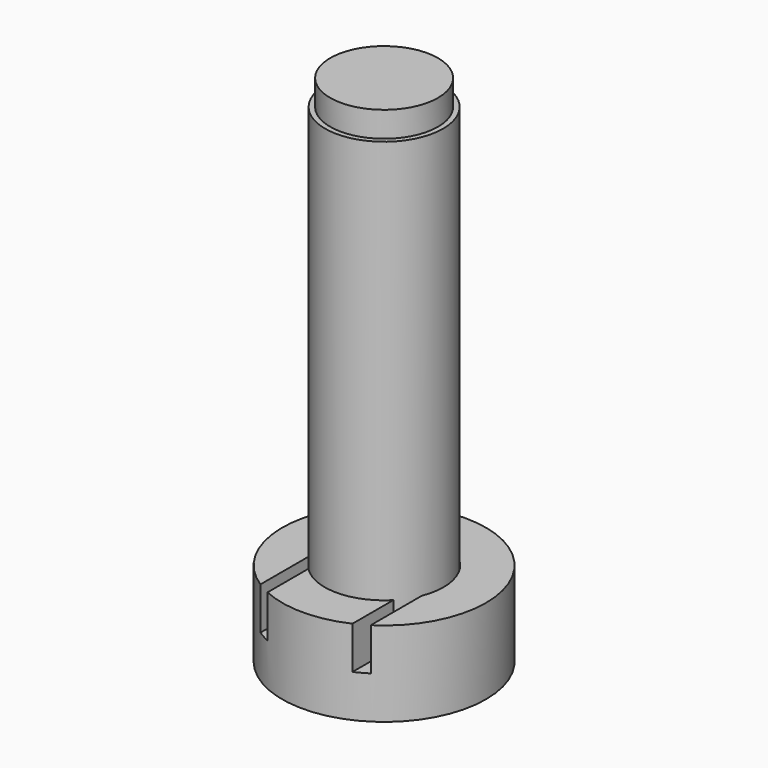
from build123d import *

# Parameters (mm, degrees)
F0_R      = 13.9
F0_R_2    = 8.7
F1_DEPTH  = 51.5
F2_R      = 12.7
F3_DEPTH  = 6
F4_R      = 10.3
F4_R_2    = 5.8
F5_DEPTH  = 2.05
F6_R      = 12.7
F7_DEPTH  = 6
F10_W     = 3
F10_H     = 25
F11_DEPTH = 10


with BuildPart() as f1:
    # F0 (on Top) → F1 (new body, symmetric)
    with BuildSketch(Plane.XY):
        Circle(F0_R)
        Circle(F0_R_2, mode=Mode.SUBTRACT)
    extrude(amount=F1_DEPTH, both=True)


with BuildPart() as f3:
    # F2 (on face) → F3 (new body)
    with BuildSketch(Plane.XY.offset(51.5)):
        Circle(F2_R)
    extrude(amount=F3_DEPTH)


with BuildPart() as f5:
    # F4 (on face) → F5 (new body)
    with BuildSketch(Plane(origin=(0, 0, -51.5), x_dir=(1, 0, 0), z_dir=(0, 0, -1))):
        Circle(F4_R)
        Circle(F4_R_2, mode=Mode.SUBTRACT)
    extrude(amount=F5_DEPTH)


with BuildPart() as f7:
    # F6 (on face) → F7 (new body)
    with BuildSketch(Plane(origin=(0, 0, -53.55), x_dir=(1, 0, 0), z_dir=(0, 0, -1))):
        Circle(F6_R)
    extrude(amount=F7_DEPTH)


with BuildPart() as f9:
    # F8 (on Front) → F9 (revolve)
    with BuildSketch(Plane.XZ):
        Polygon((5.7, -53.55), (5.7, -43.55), (0, -43.55), (0, -63.55), (24, -63.55), (24, -43.55), (14, -43.55), (14, -53.55), align=None)
    revolve(axis=Axis((0, 0, -0.0817538239), (0, 0, -1)))

    # F10 (on face) → F11 (cut, through all)
    with BuildSketch(Plane.XY.offset(-53.55)):
        with Locations((-11.5, -12.5)):
            Rectangle(F10_W, F10_H)
        with Locations((11.5, -12.5)):
            Rectangle(F10_W, F10_H)
    extrude(amount=F11_DEPTH, mode=Mode.SUBTRACT)


solid = Compound([f1.part, f3.part, f5.part, f7.part, f9.part])
